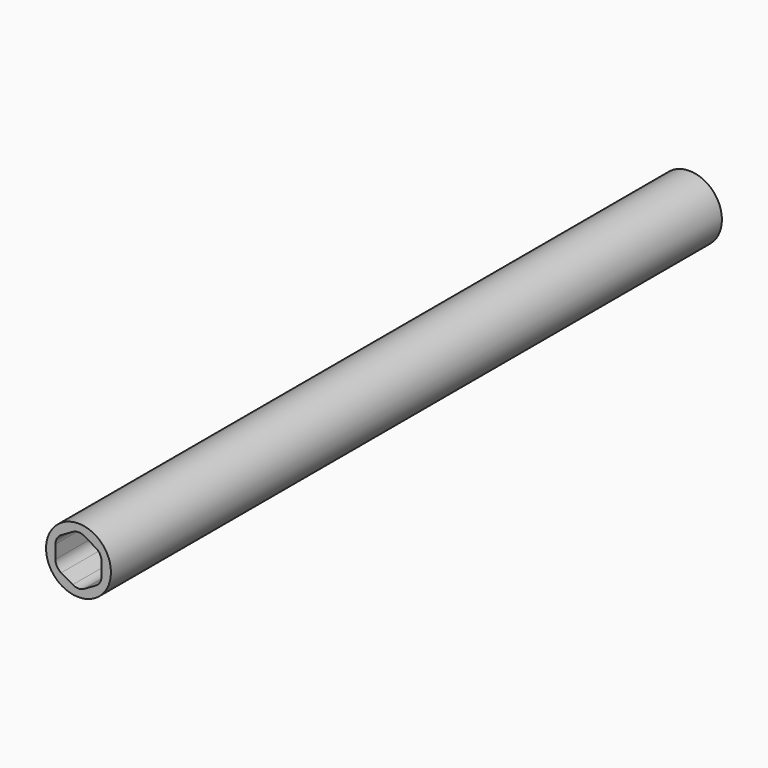
from build123d import *

# Parameters (mm, degrees)
F0_R     = 4.25
F1_DEPTH = 100


# Not quite as in the source:
# - a feature of the source that left no trace in its solid (it failed there, or was rolled back) is left out


with BuildPart() as f1:
    # F0 (on Front) → F1 (new body)
    with BuildSketch(Plane.XZ):
        Circle(F0_R)
        with BuildLine():
            ThreePointArc((2.265, 2.1737237635), (2.8140381057, 1.6246856578), (3.015, 0.8746856578))
            Line((3.015, 0.8746856578), (3.015, -0.8746856578))
            ThreePointArc((3.015, -0.8746856578), (2.8140381057, -1.6246856578), (2.265, -2.1737237635))
            Line((2.265, -2.1737237635), (0.75, -3.0484094213))
            ThreePointArc((0.75, -3.0484094213), (0, -3.2493713156), (-0.75, -3.0484094213))
            Line((-0.75, -3.0484094213), (-2.265, -2.1737237635))
            ThreePointArc((-2.265, -2.1737237635), (-2.8140381057, -1.6246856578), (-3.015, -0.8746856578))
            Line((-3.015, -0.8746856578), (-3.015, 0.8746856578))
            ThreePointArc((-3.015, 0.8746856578), (-2.8140381057, 1.6246856578), (-2.265, 2.1737237635))
            Line((-2.265, 2.1737237635), (-0.75, 3.0484094213))
            ThreePointArc((-0.75, 3.0484094213), (0, 3.2493713156), (0.75, 3.0484094213))
            Line((0.75, 3.0484094213), (2.265, 2.1737237635))
        make_face(mode=Mode.SUBTRACT)
    extrude(amount=F1_DEPTH)


solid = f1.part
